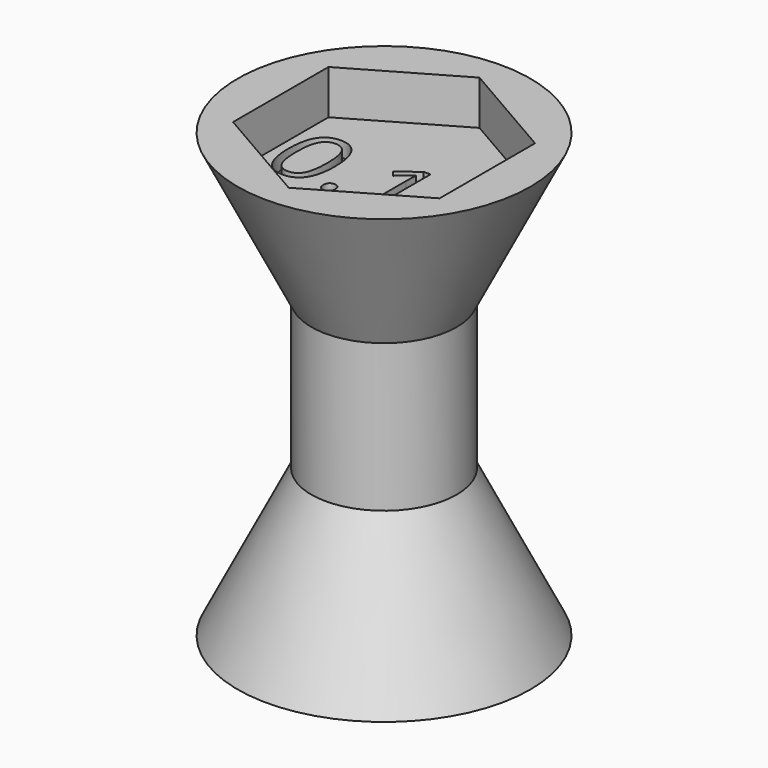
from build123d import *

# Parameters (mm, degrees)
F3_DEPTH     = 3
F4_TEXT_SIZE = 6.7887169011
F5_DEPTH     = 1


# Not quite as in the source:
# - Text() gives the source's letters only with a copy of the font that has no kerning and outlines rounded to 1/6400 em; it was checked with that copy


with BuildPart() as f1:
    # F0 (on Front) → F1 (revolve)
    with BuildSketch(Plane.XZ):
        Polygon((9.925, 15), (0, 15), (0, -15), (9.925, -15), (4.925, -5), (4.925, 5), align=None)
    revolve(axis=Axis((0, 0, 0), (0, 0, -1)))

    # F2 (on face) → F3 (cut)
    with BuildSketch(Plane.XY.offset(15)):
        Polygon((7, 4.0414518843), (0, 8.0829037687), (-7, 4.0414518843), (-7, -4.0414518843), (0, -8.0829037687), (7, -4.0414518843), align=None)
    extrude(amount=-F3_DEPTH, mode=Mode.SUBTRACT)

    # F4 (on face) → F5 (cut)
    with BuildSketch(Plane.XY.offset(12)):
        with Locations((-6.75, -2.5414518843)):
            Text('0.15', F4_TEXT_SIZE, font='Open Sans', text_align=(TextAlign.LEFT, TextAlign.BOTTOM))
    extrude(amount=-F5_DEPTH, mode=Mode.SUBTRACT)


solid = f1.part
